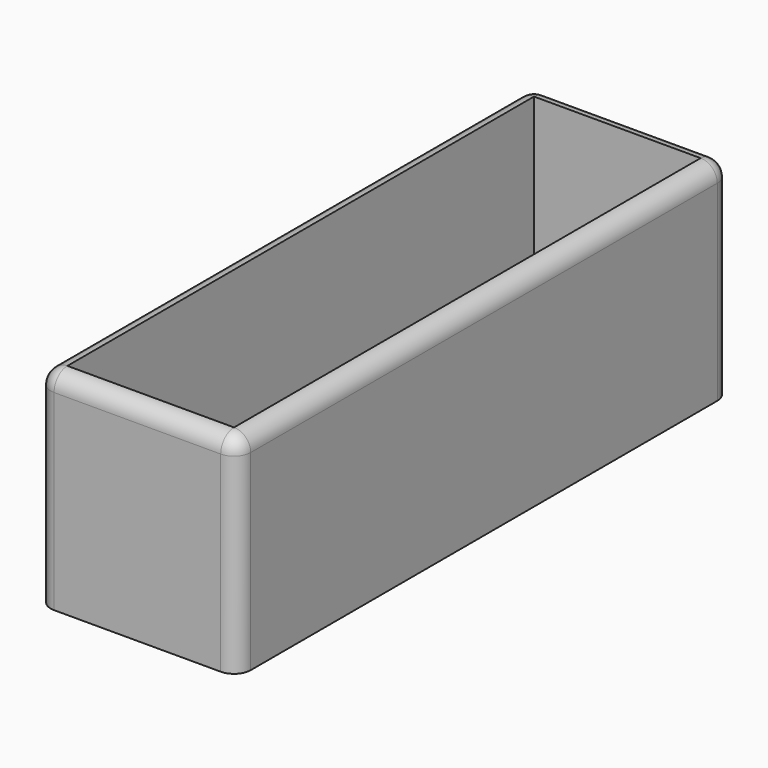
from build123d import *

# Parameters (mm, degrees)
F0_W     = 24
F0_H     = 74
F0_W_2   = 20
F0_H_2   = 70
F1_DEPTH = 25
F2_R     = 2
F3_R     = 1.99999


# Not quite as in the source:
# - a fillet or chamfer is up to 0.001 mm smaller than in the source, because OpenCascade refuses the exact size


with BuildPart() as f1:
    # F0 (on Top) → F1 (new body)
    with BuildSketch(Plane.XY):
        Rectangle(F0_W, F0_H)
        Rectangle(F0_W_2, F0_H_2, mode=Mode.SUBTRACT)
    extrude(amount=F1_DEPTH)

    # F2
    f2_edges = [f1.edges().sort_by_distance(p)[0] for p in [
        (-12, -37, 12.5),
        (12, -37, 12.5),
        (12, 37, 12.5),
        (-12, 37, 12.5),
    ]]
    fillet(f2_edges, radius=F2_R)

    # F3 (radius 2 in the source; OpenCascade refuses exactly that, so slightly less here)
    f3_edges = [f1.edges().sort_by_distance(p)[0] for p in [
        (-12, 0, 25),
    ]]
    fillet(f3_edges, radius=F3_R)


solid = f1.part
